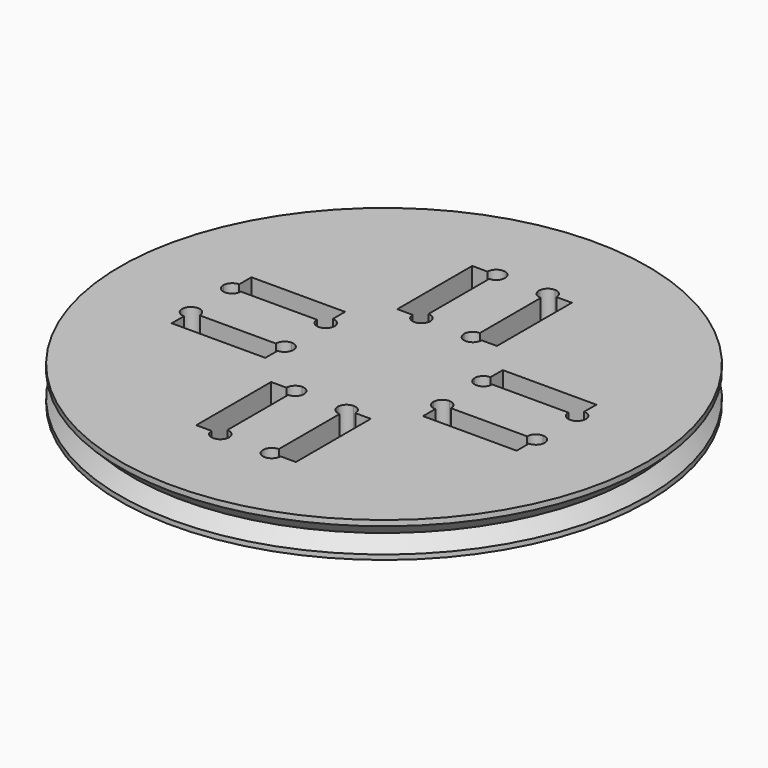
from build123d import *

# Parameters (mm, degrees)
F0_R             = 30
F0_R_2           = 6
F1_DEPTH         = 4
F2_DEPTH         = 6
F3_R             = 1.5
F4_DEPTH         = 13
F5_W             = 4.6
F5_H             = 3
F6_DEPTH         = 9.4
F11_DEPTH        = 5
F11_COPIES_COUNT = 4


# Not quite as in the source:
# - a pattern or mirror of a feature is missing from the dataset's text; its kind, count and spacing are read off the source's solid


with BuildPart() as f1:
    # F0 (on Top) → F1 (new body)
    with BuildSketch(Plane.XY):
        Circle(F0_R)
        Circle(F0_R_2, mode=Mode.SUBTRACT)
        Circle(F0_R_2)
    extrude(amount=F1_DEPTH)

    # F0 (on Top) → F2 (join)
    with BuildSketch(Plane.XY):
        Circle(F0_R_2)
    extrude(amount=-F2_DEPTH)

    # F3 (on Front) → F4 (cut, symmetric)
    with BuildSketch(Plane.XZ):
        with Locations((0, -3)):
            Circle(F3_R)
    extrude(amount=F4_DEPTH, both=True, mode=Mode.SUBTRACT)

    # F5 (on face) → F6 (cut)
    with BuildSketch(Plane(origin=(0, 0, -6), x_dir=(1, 0, 0), z_dir=(0, 0, -1))):
        with BuildLine():
            ThreePointArc((2.3, -1.5), (2.7459060435, 0), (2.3, 1.5))
            Line((2.3, 1.5), (2.3, -1.5))
        make_face()
        Rectangle(F5_W, F5_H)
        with BuildLine():
            Line((-2.3, -1.5), (-2.3, 1.5))
            ThreePointArc((-2.3, 1.5), (-2.7459060435, 0), (-2.3, -1.5))
        make_face()
    extrude(amount=-F6_DEPTH, mode=Mode.SUBTRACT)

    # F7 (on Front) → F9 (revolve, cut)
    with BuildSketch(Plane.XZ):
        Polygon((-30, 3.3777931239), (-30, 0.5493659992), (-28.5857864376, 1.9635795616), align=None)
    revolve(axis=Axis((0, 0, -3.6810841411), (0, 0, 1)), mode=Mode.SUBTRACT)

    # F10 (on face) → F11 (cut, symmetric)
    with BuildSketch(Plane.XY):
        with BuildLine():
            Line((5.6645294234, 8.9638868584), (5.6645294234, 19.6055186455))
            Line((5.6645294234, 19.6055186455), (3.9258744954, 19.6055186455))
            ThreePointArc((3.9258744954, 19.6055186455), (3.6329812765, 18.8984118643), (2.9258744954, 18.6055186455))
            Line((2.9258744954, 18.6055186455), (2.9258744954, 9.9638868584))
            ThreePointArc((2.9258744954, 9.9638868584), (3.6329812765, 9.6709936396), (3.9258744954, 8.9638868584))
            Line((3.9258744954, 8.9638868584), (5.6645294234, 8.9638868584))
        make_face()
        with BuildLine():
            Line((-2.9258744954, 9.9638868584), (-2.9258744954, 18.6055186455))
            ThreePointArc((-2.9258744954, 18.6055186455), (-3.6329812765, 18.8984118643), (-3.9258744954, 19.6055186455))
            Line((-3.9258744954, 19.6055186455), (-5.6645294234, 19.6055186455))
            Line((-5.6645294234, 19.6055186455), (-5.6645294234, 8.9638868584))
            Line((-5.6645294234, 8.9638868584), (-3.9258744954, 8.9638868584))
            ThreePointArc((-3.9258744954, 8.9638868584), (-3.6329812765, 9.6709936396), (-2.9258744954, 9.9638868584))
        make_face()
        with BuildLine():
            ThreePointArc((2.9258744954, 18.6055186455), (3.6329812765, 18.8984118643), (3.9258744954, 19.6055186455))
            Line((3.9258744954, 19.6055186455), (2.9258744954, 19.6055186455))
            Line((2.9258744954, 19.6055186455), (2.9258744954, 18.6055186455))
        make_face()
        with BuildLine():
            Line((2.9258744954, 18.6055186455), (2.9258744954, 19.6055186455))
            Line((2.9258744954, 19.6055186455), (1.9258744954, 19.6055186455))
            ThreePointArc((1.9258744954, 19.6055186455), (2.2187677142, 18.8984118643), (2.9258744954, 18.6055186455))
        make_face()
        with BuildLine():
            Line((-2.9258744954, 18.6055186455), (-2.9258744954, 19.6055186455))
            Line((-2.9258744954, 19.6055186455), (-3.9258744954, 19.6055186455))
            ThreePointArc((-3.9258744954, 19.6055186455), (-3.6329812765, 18.8984118643), (-2.9258744954, 18.6055186455))
        make_face()
        with BuildLine():
            Line((2.9258744954, 8.9638868584), (3.9258744954, 8.9638868584))
            ThreePointArc((3.9258744954, 8.9638868584), (3.6329812765, 9.6709936396), (2.9258744954, 9.9638868584))
            Line((2.9258744954, 9.9638868584), (2.9258744954, 8.9638868584))
        make_face()
        with BuildLine():
            ThreePointArc((-2.9258744954, 18.6055186455), (-2.2187677142, 18.8984118643), (-1.9258744954, 19.6055186455))
            Line((-1.9258744954, 19.6055186455), (-2.9258744954, 19.6055186455))
            Line((-2.9258744954, 19.6055186455), (-2.9258744954, 18.6055186455))
        make_face()
        with BuildLine():
            Line((-2.9258744954, 8.9638868584), (-2.9258744954, 9.9638868584))
            ThreePointArc((-2.9258744954, 9.9638868584), (-3.6329812765, 9.6709936396), (-3.9258744954, 8.9638868584))
            Line((-3.9258744954, 8.9638868584), (-2.9258744954, 8.9638868584))
        make_face()
        with BuildLine():
            Line((2.9258744954, 8.9638868584), (2.9258744954, 9.9638868584))
            ThreePointArc((2.9258744954, 9.9638868584), (2.2187677142, 9.6709936396), (1.9258744954, 8.9638868584))
            Line((1.9258744954, 8.9638868584), (2.9258744954, 8.9638868584))
        make_face()
        with BuildLine():
            Line((-2.9258744954, 8.9638868584), (-1.9258744954, 8.9638868584))
            ThreePointArc((-1.9258744954, 8.9638868584), (-2.2187677142, 9.6709936396), (-2.9258744954, 9.9638868584))
            Line((-2.9258744954, 9.9638868584), (-2.9258744954, 8.9638868584))
        make_face()
        with BuildLine():
            Line((2.9258744954, 19.6055186455), (3.9258744954, 19.6055186455))
            ThreePointArc((3.9258744954, 19.6055186455), (3.6329812765, 20.3126254267), (2.9258744954, 20.6055186455))
            Line((2.9258744954, 20.6055186455), (2.9258744954, 19.6055186455))
        make_face()
        with BuildLine():
            Line((1.9258744954, 19.6055186455), (2.9258744954, 19.6055186455))
            Line((2.9258744954, 19.6055186455), (2.9258744954, 20.6055186455))
            ThreePointArc((2.9258744954, 20.6055186455), (2.2187677142, 20.3126254267), (1.9258744954, 19.6055186455))
        make_face()
        with BuildLine():
            Line((-2.9258744954, 19.6055186455), (-1.9258744954, 19.6055186455))
            ThreePointArc((-1.9258744954, 19.6055186455), (-2.2187677142, 20.3126254267), (-2.9258744954, 20.6055186455))
            Line((-2.9258744954, 20.6055186455), (-2.9258744954, 19.6055186455))
        make_face()
        with BuildLine():
            Line((-3.9258744954, 19.6055186455), (-2.9258744954, 19.6055186455))
            Line((-2.9258744954, 19.6055186455), (-2.9258744954, 20.6055186455))
            ThreePointArc((-2.9258744954, 20.6055186455), (-3.6329812765, 20.3126254267), (-3.9258744954, 19.6055186455))
        make_face()
        with BuildLine():
            ThreePointArc((-2.9258744954, 7.9638868584), (-2.2187677142, 8.2567800773), (-1.9258744954, 8.9638868584))
            Line((-1.9258744954, 8.9638868584), (-2.9258744954, 8.9638868584))
            Line((-2.9258744954, 8.9638868584), (-2.9258744954, 7.9638868584))
        make_face()
        with BuildLine():
            Line((2.9258744954, 7.9638868584), (2.9258744954, 8.9638868584))
            Line((2.9258744954, 8.9638868584), (1.9258744954, 8.9638868584))
            ThreePointArc((1.9258744954, 8.9638868584), (2.2187677142, 8.2567800773), (2.9258744954, 7.9638868584))
        make_face()
        with BuildLine():
            ThreePointArc((2.9258744954, 7.9638868584), (3.6329812765, 8.2567800773), (3.9258744954, 8.9638868584))
            Line((3.9258744954, 8.9638868584), (2.9258744954, 8.9638868584))
            Line((2.9258744954, 8.9638868584), (2.9258744954, 7.9638868584))
        make_face()
        with BuildLine():
            Line((-2.9258744954, 7.9638868584), (-2.9258744954, 8.9638868584))
            Line((-2.9258744954, 8.9638868584), (-3.9258744954, 8.9638868584))
            ThreePointArc((-3.9258744954, 8.9638868584), (-3.6329812765, 8.2567800773), (-2.9258744954, 7.9638868584))
        make_face()
    f11 = extrude(amount=F11_DEPTH, both=True, mode=Mode.SUBTRACT)

    # F11_copies: F11 ×4 about axis
    f11_copies_axis = Axis((0, 0, 0), (0, 0, 1))
    for i in range(1, F11_COPIES_COUNT):
        add(f11.rotate(f11_copies_axis, i * 360 / F11_COPIES_COUNT), mode=Mode.SUBTRACT)


solid = f1.part
